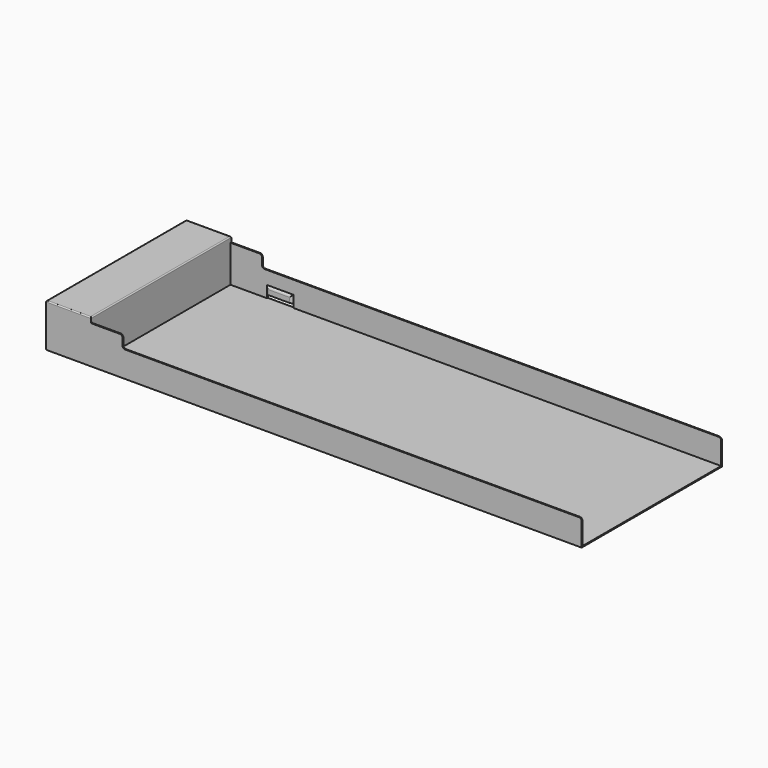
from build123d import *

# Parameters (mm, degrees)
F0_W          = 52
F0_H          = 1.2
F0_H_2        = 200.6
F1_DEPTH      = 50
F0_W_2        = 36.4451892475
F2_DEPTH      = 44
F0_W_3        = 531.5548107525
F3_DEPTH      = 30
F4_DEPTH      = 1.2
F5_R          = 1.2
F6_R          = 3
F7_W          = 30.6323694531
F7_H          = 5.0316524575
F8_DEPTH      = 25
F9_W          = 30.6323694531
F9_H          = 8.4860329516
F10_DEPTH     = 2
F11_T1_DEPTH  = 44.7745050768
F11_T6_DEPTH  = 22.6281685754
F11_T11_DEPTH = 22.6281685754


# Not quite as in the source:
# - a fillet or chamfer that OpenCascade refuses, or shapes differently, is made with other operations: its cross-section is extruded or revolved along the edge and cut away or added


with BuildPart() as f1:
    # F0 (on Top) → F1 (new body)
    with BuildSketch(Plane.XY):
        with Locations((-71.6174369702, 163.7731539965)):
            Rectangle(F0_W, F0_H)
        with Locations((-71.6174369702, 62.8731539965)):
            Rectangle(F0_W, F0_H_2)
        with Locations((-71.6174369702, -38.0268460035)):
            Rectangle(F0_W, F0_H)
    extrude(amount=F1_DEPTH)

    # F0 (on Top) → F2 (join)
    with BuildSketch(Plane.XY):
        with Locations((-27.3948423465, -38.0268460035)):
            Rectangle(F0_W_2, F0_H)
        with Locations((-27.3948423465, 163.7731539965)):
            Rectangle(F0_W_2, F0_H)
    extrude(amount=F2_DEPTH)

    # F0 (on Top) → F3 (join)
    with BuildSketch(Plane.XY):
        with Locations((256.6051576535, 163.7731539965)):
            Rectangle(F0_W_3, F0_H)
        with Locations((256.6051576535, -38.0268460035)):
            Rectangle(F0_W_3, F0_H)
    extrude(amount=F3_DEPTH)

    # F0 (on Top) → F4 (join)
    with BuildSketch(Plane.XY):
        with Locations((256.6051576535, 62.8731539965)):
            Rectangle(F0_W_3, F0_H_2)
        with Locations((-27.3948423465, 62.8731539965)):
            Rectangle(F0_W_2, F0_H_2)
    extrude(amount=F4_DEPTH)

    # F5
    f5_edges = [f1.edges().sort_by_distance(p)[0] for p in [
        (-71.617437, -38.626846, 50),
        (-71.617437, 164.373154, 50),
        (-97.617437, 62.873154, 50),
        (-97.617437, 62.873154, 0),
        (-45.617437, 62.873154, 50),
        (-45.617437, -38.026846, 44),
    ]]
    fillet(f5_edges, radius=F5_R)

    # F6
    f6_edges = [f1.edges().sort_by_distance(p)[0] for p in [
        (-9.172248, -38.026846, 44),
        (522.382563, -38.026846, 30),
        (522.382563, 163.773154, 30),
        (-9.172248, 163.773154, 44),
        (-9.172248, 163.773154, 30),
        (-9.172248, -38.026846, 30),
    ]]
    fillet(f6_edges, radius=F6_R)

    # F7 (on face) → F8 (cut)
    with BuildSketch(Plane.XZ.offset(-163.1731539965)):
        with Locations((11.9725436671, 3.6928627233)):
            Rectangle(F7_W, F7_H)
    extrude(amount=-F8_DEPTH, mode=Mode.SUBTRACT)

    # F9 (on face) → F10 (join)
    with BuildSketch(Plane.XZ.offset(-163.1731539965)):
        with Locations((11.9725436671, 10.4517054278)):
            Rectangle(F9_W, F9_H)
    extrude(amount=F10_DEPTH)

    # F11: fillet of radius 3 on 3 edges, made by hand

    # F11_s2 → F11_t1 (cut)
    with BuildSketch(Plane.YZ.offset(-10.4147088713)):
        with BuildLine():
            ThreePointArc((163.1731539965, 14.6947219037), (161.7236642537, 13.5983455865), (161.1731539965, 11.8662947789))
            Line((161.1731539965, 11.8662947789), (161.1731539965, 14.6947219037))
            Line((161.1731539965, 14.6947219037), (163.1731539965, 14.6947219037))
        make_face()
    extrude(amount=F11_T1_DEPTH, mode=Mode.SUBTRACT)


with BuildPart() as f11_tool4:
    # F11_s5 → F11_t6 (new body)
    with BuildSketch(Plane.XY.offset(-0.8623788598)):
        with BuildLine():
            ThreePointArc((27.2887283936, 163.1731539965), (26.1923520764, 161.7236642537), (24.4603012689, 161.1731539965))
            Line((24.4603012689, 161.1731539965), (27.2887283936, 161.1731539965))
            Line((27.2887283936, 161.1731539965), (27.2887283936, 163.1731539965))
        make_face()
    extrude(amount=F11_T6_DEPTH)

    split(bisect_by=Plane.XY.offset(1.2), keep=Keep.TOP)


with BuildPart() as f1_1:
    add(f1.part)

    # F11_t3: cut F11_tool4
    add(f11_tool4.part, mode=Mode.SUBTRACT)


with BuildPart() as f11_tool9:
    # F11_s10 → F11_t11 (new body)
    with BuildSketch(Plane.XY.offset(21.7657897155)):
        with BuildLine():
            ThreePointArc((-3.3436410595, 163.1731539965), (-2.2472647423, 161.7236642537), (-0.5152139347, 161.1731539965))
            Line((-0.5152139347, 161.1731539965), (-3.3436410595, 161.1731539965))
            Line((-3.3436410595, 161.1731539965), (-3.3436410595, 163.1731539965))
        make_face()
    extrude(amount=-F11_T11_DEPTH)

    split(bisect_by=Plane.XY.offset(1.2), keep=Keep.TOP)


with BuildPart() as f1_2:
    add(f1_1.part)

    # F11_t8: cut F11_tool9
    add(f11_tool9.part, mode=Mode.SUBTRACT)


solid = f1_2.part
